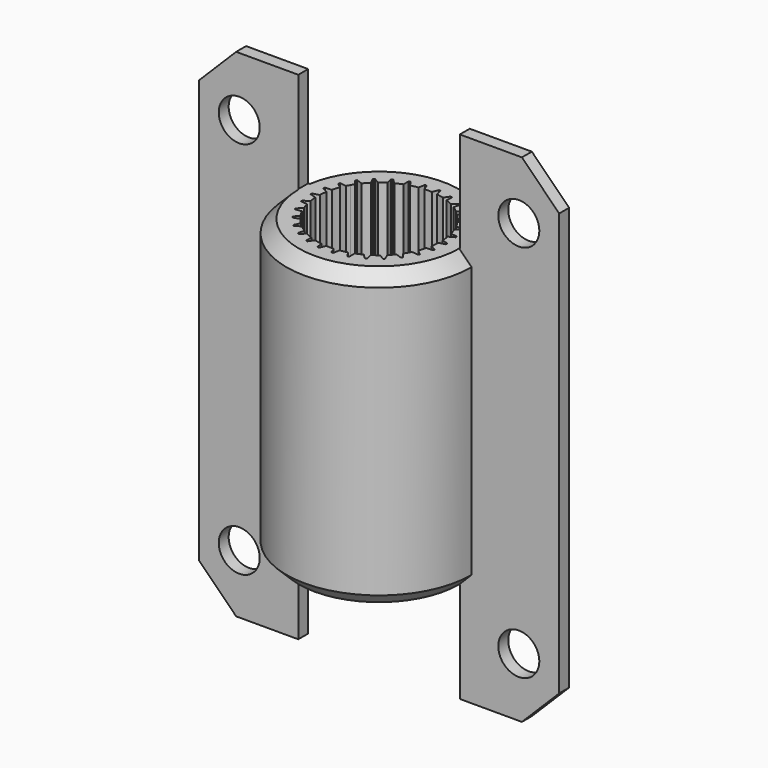
from build123d import *

# Parameters (mm, degrees)
F0_R         = 7.45
F1_DEPTH     = 11.9
F2_R         = 1.65
F3_DEPTH     = 1
F4_T2_ANGLE  = 180
F4_T6_ANGLE  = 204.1813114707
F4_T9_ANGLE  = 180
F4_T13_ANGLE = 204.1813114707
F5_SIZE      = 3


# Not quite as in the source:
# - a fillet or chamfer that OpenCascade refuses, or shapes differently, is made with other operations: its cross-section is extruded or revolved along the edge and cut away or added


with BuildPart() as f1:
    # F0 (on Top) → F1 (new body, symmetric)
    with BuildSketch(Plane.XY):
        Circle(F0_R)
        with BuildLine():
            ThreePointArc((5.449550226, 0.0700166693), (5.4498875553, 0.0350090569), (5.45, 0))
            ThreePointArc((5.45, 0), (5.4498875553, -0.0350090569), (5.449550226, -0.0700166693))
            ThreePointArc((5.449550226, -0.0700166693), (5.4201443298, -0.5696801248), (5.3450217628, -1.0645385646))
            ThreePointArc((5.3450217628, -1.0645385646), (5.330904424, -1.133118715), (5.3159071946, -1.2015118387))
            ThreePointArc((5.3159071946, -1.2015118387), (5.1832580138, -1.6841426193), (5.0068902002, -2.152568355))
            ThreePointArc((5.0068902002, -2.152568355), (4.9788227442, -2.2167147048), (4.9499335102, -2.2804951754))
            ThreePointArc((4.9499335102, -2.2804951754), (4.7198384506, -2.725), (4.4499335102, -3.1465205792))
            ThreePointArc((4.4499335102, -3.1465205792), (4.4091426193, -3.203429625), (4.3676239789, -3.2598099298))
            ThreePointArc((4.3676239789, -3.2598099298), (4.0501392989, -3.6467618047), (3.6984933726, -4.0029547553))
            ThreePointArc((3.6984933726, -4.0029547553), (3.6467618047, -4.0501392989), (3.5944283217, -4.096655348))
            ThreePointArc((3.5944283217, -4.096655348), (3.203429625, -4.4091426193), (2.7854113273, -4.6844406003))
            ThreePointArc((2.7854113273, -4.6844406003), (2.725, -4.7198384506), (2.6641388987, -4.7544572696))
            ThreePointArc((2.6641388987, -4.7544572696), (2.2167147048, -4.9788227442), (1.7505934411, -5.1611939127))
            ThreePointArc((1.7505934411, -5.1611939127), (1.6841426193, -5.1832580138), (1.617413822, -5.204466594))
            ThreePointArc((1.617413822, -5.204466594), (1.133118715, -5.330904424), (0.6392662213, -5.4123782849))
            ThreePointArc((0.6392662213, -5.4123782849), (0.5696801248, -5.4201443298), (0.5, -5.4270157545))
            ThreePointArc((0.5, -5.4270157545), (0, -5.45), (-0.5, -5.4270157545))
            ThreePointArc((-0.5, -5.4270157545), (-0.5696801248, -5.4201443298), (-0.6392662213, -5.4123782849))
            ThreePointArc((-0.6392662213, -5.4123782849), (-1.133118715, -5.330904424), (-1.617413822, -5.204466594))
            ThreePointArc((-1.617413822, -5.204466594), (-1.6841426193, -5.1832580138), (-1.7505934411, -5.1611939127))
            ThreePointArc((-1.7505934411, -5.1611939127), (-2.2167147048, -4.9788227442), (-2.6641388987, -4.7544572696))
            ThreePointArc((-2.6641388987, -4.7544572696), (-2.725, -4.7198384506), (-2.7854113273, -4.6844406003))
            ThreePointArc((-2.7854113273, -4.6844406003), (-3.203429625, -4.4091426193), (-3.5944283217, -4.096655348))
            ThreePointArc((-3.5944283217, -4.096655348), (-3.6467618047, -4.0501392989), (-3.6984933726, -4.0029547553))
            ThreePointArc((-3.6984933726, -4.0029547553), (-4.0501392989, -3.6467618047), (-4.3676239789, -3.2598099298))
            ThreePointArc((-4.3676239789, -3.2598099298), (-4.4091426193, -3.203429625), (-4.4499335102, -3.1465205792))
            ThreePointArc((-4.4499335102, -3.1465205792), (-4.7198384506, -2.725), (-4.9499335102, -2.2804951754))
            ThreePointArc((-4.9499335102, -2.2804951754), (-4.9788227442, -2.2167147048), (-5.0068902002, -2.152568355))
            ThreePointArc((-5.0068902002, -2.152568355), (-5.1832580138, -1.6841426193), (-5.3159071946, -1.2015118387))
            ThreePointArc((-5.3159071946, -1.2015118387), (-5.330904424, -1.133118715), (-5.3450217628, -1.0645385646))
            ThreePointArc((-5.3450217628, -1.0645385646), (-5.4201443298, -0.5696801248), (-5.449550226, -0.0700166693))
            ThreePointArc((-5.449550226, -0.0700166693), (-5.45, 0), (-5.449550226, 0.0700166693))
            ThreePointArc((-5.449550226, 0.0700166693), (-5.4201443298, 0.5696801248), (-5.3450217628, 1.0645385646))
            ThreePointArc((-5.3450217628, 1.0645385646), (-5.330904424, 1.133118715), (-5.3159071946, 1.2015118387))
            ThreePointArc((-5.3159071946, 1.2015118387), (-5.1832580138, 1.6841426193), (-5.0068902002, 2.152568355))
            ThreePointArc((-5.0068902002, 2.152568355), (-4.9788227442, 2.2167147048), (-4.9499335102, 2.2804951754))
            ThreePointArc((-4.9499335102, 2.2804951754), (-4.7198384506, 2.725), (-4.4499335102, 3.1465205792))
            ThreePointArc((-4.4499335102, 3.1465205792), (-4.4091426193, 3.203429625), (-4.3676239789, 3.2598099298))
            ThreePointArc((-4.3676239789, 3.2598099298), (-4.0501392989, 3.6467618047), (-3.6984933726, 4.0029547553))
            ThreePointArc((-3.6984933726, 4.0029547553), (-3.6467618047, 4.0501392989), (-3.5944283217, 4.096655348))
            ThreePointArc((-3.5944283217, 4.096655348), (-3.203429625, 4.4091426193), (-2.7854113273, 4.6844406003))
            ThreePointArc((-2.7854113273, 4.6844406003), (-2.725, 4.7198384506), (-2.6641388987, 4.7544572696))
            ThreePointArc((-2.6641388987, 4.7544572696), (-2.2167147048, 4.9788227442), (-1.7505934411, 5.1611939127))
            ThreePointArc((-1.7505934411, 5.1611939127), (-1.6841426193, 5.1832580138), (-1.617413822, 5.204466594))
            ThreePointArc((-1.617413822, 5.204466594), (-1.133118715, 5.330904424), (-0.6392662213, 5.4123782849))
            ThreePointArc((-0.6392662213, 5.4123782849), (-0.5696801248, 5.4201443298), (-0.5, 5.4270157545))
            ThreePointArc((-0.5, 5.4270157545), (0, 5.45), (0.5, 5.4270157545))
            ThreePointArc((0.5, 5.4270157545), (0.5696801248, 5.4201443298), (0.6392662213, 5.4123782849))
            ThreePointArc((0.6392662213, 5.4123782849), (1.133118715, 5.330904424), (1.617413822, 5.204466594))
            ThreePointArc((1.617413822, 5.204466594), (1.6841426193, 5.1832580138), (1.7505934411, 5.1611939127))
            ThreePointArc((1.7505934411, 5.1611939127), (2.2167147048, 4.9788227442), (2.6641388987, 4.7544572696))
            ThreePointArc((2.6641388987, 4.7544572696), (2.725, 4.7198384506), (2.7854113273, 4.6844406003))
            ThreePointArc((2.7854113273, 4.6844406003), (3.203429625, 4.4091426193), (3.5944283217, 4.096655348))
            ThreePointArc((3.5944283217, 4.096655348), (3.6467618047, 4.0501392989), (3.6984933726, 4.0029547553))
            ThreePointArc((3.6984933726, 4.0029547553), (4.0501392989, 3.6467618047), (4.3676239789, 3.2598099298))
            ThreePointArc((4.3676239789, 3.2598099298), (4.4091426193, 3.203429625), (4.4499335102, 3.1465205792))
            ThreePointArc((4.4499335102, 3.1465205792), (4.7198384506, 2.725), (4.9499335102, 2.2804951754))
            ThreePointArc((4.9499335102, 2.2804951754), (4.9788227442, 2.2167147048), (5.0068902002, 2.152568355))
            ThreePointArc((5.0068902002, 2.152568355), (5.1832580138, 1.6841426193), (5.3159071946, 1.2015118387))
            ThreePointArc((5.3159071946, 1.2015118387), (5.330904424, 1.133118715), (5.3450217628, 1.0645385646))
            ThreePointArc((5.3450217628, 1.0645385646), (5.4201443298, 0.5696801248), (5.449550226, 0.0700166693))
        make_face(mode=Mode.SUBTRACT)
        with BuildLine():
            Line((-3.471065627, 3.5290513475), (-3.6984933726, 4.0029547553))
            ThreePointArc((-3.6984933726, 4.0029547553), (-4.0501392989, 3.6467618047), (-4.3676239789, 3.2598099298))
            Line((-4.3676239789, 3.2598099298), (-3.8725439908, 3.0831644522))
            ThreePointArc((-3.8725439908, 3.0831644522), (-3.7772917267, 3.1991510141), (-3.6785668861, 3.3121965015))
            ThreePointArc((-3.6785668861, 3.3121965015), (-3.5764602296, 3.4221969882), (-3.471065627, 3.5290513475))
        make_face()
        with BuildLine():
            Line((-4.1289455477, 2.7302579849), (-4.4499335102, 3.1465205792))
            ThreePointArc((-4.4499335102, 3.1465205792), (-4.7198384506, 2.725), (-4.9499335102, 2.2804951754))
            Line((-4.9499335102, 2.2804951754), (-4.4289455477, 2.2106427427))
            ThreePointArc((-4.4289455477, 2.2106427427), (-4.3598897363, 2.3438987792), (-4.2868257487, 2.475))
            ThreePointArc((-4.2868257487, 2.475), (-4.2098207549, 2.6038258797), (-4.1289455477, 2.7302579849))
        make_face()
        with BuildLine():
            Line((-2.6614834824, 4.1736082318), (-2.7854113273, 4.6844406003))
            ThreePointArc((-2.7854113273, 4.6844406003), (-3.203429625, 4.4091426193), (-3.5944283217, 4.096655348))
            Line((-3.5944283217, 4.096655348), (-3.146893679, 3.8209370805))
            ThreePointArc((-3.146893679, 3.8209370805), (-3.0296079432, 3.9145849985), (-2.9095369988, 4.0046341222))
            ThreePointArc((-2.9095369988, 4.0046341222), (-2.7867912306, 4.0910016667), (-2.6614834824, 4.1736082318))
        make_face()
        with BuildLine():
            Line((-1.7355817384, 4.6357584093), (-1.7505934411, 5.1611939127))
            ThreePointArc((-1.7505934411, 5.1611939127), (-2.2167147048, 4.9788227442), (-2.6641388987, 4.7544572696))
            Line((-2.6641388987, 4.7544572696), (-2.283709013, 4.3917164234))
            ThreePointArc((-2.283709013, 4.3917164234), (-2.149515755, 4.4589328341), (-2.0133463832, 4.5220500153))
            ThreePointArc((-2.0133463832, 4.5220500153), (-1.8753260823, 4.5810099416), (-1.7355817384, 4.6357584093))
        make_face()
        with BuildLine():
            Line((-0.7338267442, 4.8953036994), (-0.6392662213, 5.4123782849))
            ThreePointArc((-0.6392662213, 5.4123782849), (-1.133118715, 5.330904424), (-1.617413822, 5.204466594))
            Line((-1.617413822, 5.204466594), (-1.3207153047, 4.7705566849))
            ThreePointArc((-1.3207153047, 4.7705566849), (-1.1754794137, 4.8084039086), (-1.0291628695, 4.8418306236))
            ThreePointArc((-1.0291628695, 4.8418306236), (-0.8819001854, 4.8708060999), (-0.7338267442, 4.8953036994))
        make_face()
        with BuildLine():
            Line((0.3, 4.9409007276), (0.5, 5.4270157545))
            ThreePointArc((0.5, 5.4270157545), (0, 5.45), (-0.5, 5.4270157545))
            Line((-0.5, 5.4270157545), (-0.3, 4.9409007276))
            ThreePointArc((-0.3, 4.9409007276), (-0.1500689814, 4.947724659), (0, 4.95))
            ThreePointArc((0, 4.95), (0.1500689814, 4.947724659), (0.3, 4.9409007276))
        make_face()
        with BuildLine():
            Line((1.3207153047, 4.7705566849), (1.617413822, 5.204466594))
            ThreePointArc((1.617413822, 5.204466594), (1.133118715, 5.330904424), (0.6392662213, 5.4123782849))
            Line((0.6392662213, 5.4123782849), (0.7338267442, 4.8953036994))
            ThreePointArc((0.7338267442, 4.8953036994), (0.8819001854, 4.8708060999), (1.0291628695, 4.8418306236))
            ThreePointArc((1.0291628695, 4.8418306236), (1.1754794137, 4.8084039086), (1.3207153047, 4.7705566849))
        make_face()
        with BuildLine():
            Line((2.283709013, 4.3917164234), (2.6641388987, 4.7544572696))
            ThreePointArc((2.6641388987, 4.7544572696), (2.2167147048, 4.9788227442), (1.7505934411, 5.1611939127))
            Line((1.7505934411, 5.1611939127), (1.7355817384, 4.6357584093))
            ThreePointArc((1.7355817384, 4.6357584093), (1.8753260823, 4.5810099416), (2.0133463832, 4.5220500153))
            ThreePointArc((2.0133463832, 4.5220500153), (2.149515755, 4.4589328341), (2.283709013, 4.3917164234))
        make_face()
        with BuildLine():
            Line((3.146893679, 3.8209370805), (3.5944283217, 4.096655348))
            ThreePointArc((3.5944283217, 4.096655348), (3.203429625, 4.4091426193), (2.7854113273, 4.6844406003))
            Line((2.7854113273, 4.6844406003), (2.6614834824, 4.1736082318))
            ThreePointArc((2.6614834824, 4.1736082318), (2.7867912306, 4.0910016667), (2.9095369988, 4.0046341222))
            ThreePointArc((2.9095369988, 4.0046341222), (3.0296079432, 3.9145849985), (3.146893679, 3.8209370805))
        make_face()
        with BuildLine():
            Line((3.8725439908, 3.0831644522), (4.3676239789, 3.2598099298))
            ThreePointArc((4.3676239789, 3.2598099298), (4.0501392989, 3.6467618047), (3.6984933726, 4.0029547553))
            Line((3.6984933726, 4.0029547553), (3.471065627, 3.5290513475))
            ThreePointArc((3.471065627, 3.5290513475), (3.5764602296, 3.4221969882), (3.6785668861, 3.3121965015))
            ThreePointArc((3.6785668861, 3.3121965015), (3.7772917267, 3.1991510141), (3.8725439908, 3.0831644522))
        make_face()
        with BuildLine():
            Line((4.4289455477, 2.2106427427), (4.9499335102, 2.2804951754))
            ThreePointArc((4.9499335102, 2.2804951754), (4.7198384506, 2.725), (4.4499335102, 3.1465205792))
            Line((4.4499335102, 3.1465205792), (4.1289455477, 2.7302579849))
            ThreePointArc((4.1289455477, 2.7302579849), (4.2098207549, 2.6038258797), (4.2868257487, 2.475))
            ThreePointArc((4.2868257487, 2.475), (4.3598897363, 2.3438987792), (4.4289455477, 2.2106427427))
        make_face()
        with BuildLine():
            Line((4.7917809317, 1.2415053375), (5.3159071946, 1.2015118387))
            ThreePointArc((5.3159071946, 1.2015118387), (5.1832580138, 1.6841426193), (5.0068902002, 2.152568355))
            Line((5.0068902002, 2.152568355), (4.606370735, 1.8121392472))
            ThreePointArc((4.606370735, 1.8121392472), (4.6591919121, 1.6716550858), (4.7077297557, 1.5296341222))
            ThreePointArc((4.7077297557, 1.5296341222), (4.7519396433, 1.3862069204), (4.7917809317, 1.2415053375))
        make_face()
        with BuildLine():
            Line((4.9451924954, 0.2181081916), (5.449550226, 0.0700166693))
            ThreePointArc((5.449550226, 0.0700166693), (5.4201443298, 0.5696801248), (5.3450217628, 1.0645385646))
            Line((5.3450217628, 1.0645385646), (4.8824754175, 0.8148213288))
            ThreePointArc((4.8824754175, 0.8148213288), (4.9049340256, 0.6664249431), (4.9228833821, 0.5174158932))
            ThreePointArc((4.9228833821, 0.5174158932), (4.9363069856, 0.3679311674), (4.9451924954, 0.2181081916))
        make_face()
        with BuildLine():
            Line((-4.606370735, 1.8121392472), (-5.0068902002, 2.152568355))
            ThreePointArc((-5.0068902002, 2.152568355), (-5.1832580138, 1.6841426193), (-5.3159071946, 1.2015118387))
            Line((-5.3159071946, 1.2015118387), (-4.7917809317, 1.2415053375))
            ThreePointArc((-4.7917809317, 1.2415053375), (-4.7519396433, 1.3862069204), (-4.7077297557, 1.5296341222))
            ThreePointArc((-4.7077297557, 1.5296341222), (-4.6591919121, 1.6716550858), (-4.606370735, 1.8121392472))
        make_face()
        with BuildLine():
            Line((-4.8824754175, 0.8148213288), (-5.3450217628, 1.0645385646))
            ThreePointArc((-5.3450217628, 1.0645385646), (-5.4201443298, 0.5696801248), (-5.449550226, 0.0700166693))
            Line((-5.449550226, 0.0700166693), (-4.9451924954, 0.2181081916))
            ThreePointArc((-4.9451924954, 0.2181081916), (-4.9363069856, 0.3679311674), (-4.9228833821, 0.5174158932))
            ThreePointArc((-4.9228833821, 0.5174158932), (-4.9049340256, 0.6664249431), (-4.8824754175, 0.8148213288))
        make_face()
        with BuildLine():
            ThreePointArc((-5.449550226, -0.0700166693), (-5.4201443298, -0.5696801248), (-5.3450217628, -1.0645385646))
            Line((-5.3450217628, -1.0645385646), (-4.8824754175, -0.8148213288))
            ThreePointArc((-4.8824754175, -0.8148213288), (-4.9049340256, -0.6664249431), (-4.9228833821, -0.5174158932))
            ThreePointArc((-4.9228833821, -0.5174158932), (-4.9363069856, -0.3679311674), (-4.9451924954, -0.2181081916))
            Line((-4.9451924954, -0.2181081916), (-5.449550226, -0.0700166693))
        make_face()
        with BuildLine():
            ThreePointArc((-5.3159071946, -1.2015118387), (-5.1832580138, -1.6841426193), (-5.0068902002, -2.152568355))
            Line((-5.0068902002, -2.152568355), (-4.606370735, -1.8121392472))
            ThreePointArc((-4.606370735, -1.8121392472), (-4.6591919121, -1.6716550858), (-4.7077297557, -1.5296341222))
            ThreePointArc((-4.7077297557, -1.5296341222), (-4.7519396433, -1.3862069204), (-4.7917809317, -1.2415053375))
            Line((-4.7917809317, -1.2415053375), (-5.3159071946, -1.2015118387))
        make_face()
        with BuildLine():
            ThreePointArc((-4.9499335102, -2.2804951754), (-4.7198384506, -2.725), (-4.4499335102, -3.1465205792))
            Line((-4.4499335102, -3.1465205792), (-4.1289455477, -2.7302579849))
            ThreePointArc((-4.1289455477, -2.7302579849), (-4.2098207549, -2.6038258797), (-4.2868257487, -2.475))
            ThreePointArc((-4.2868257487, -2.475), (-4.3598897363, -2.3438987792), (-4.4289455477, -2.2106427427))
            Line((-4.4289455477, -2.2106427427), (-4.9499335102, -2.2804951754))
        make_face()
        with BuildLine():
            ThreePointArc((-4.3676239789, -3.2598099298), (-4.0501392989, -3.6467618047), (-3.6984933726, -4.0029547553))
            Line((-3.6984933726, -4.0029547553), (-3.471065627, -3.5290513475))
            ThreePointArc((-3.471065627, -3.5290513475), (-3.5764602296, -3.4221969882), (-3.6785668861, -3.3121965015))
            ThreePointArc((-3.6785668861, -3.3121965015), (-3.7772917267, -3.1991510141), (-3.8725439908, -3.0831644522))
            Line((-3.8725439908, -3.0831644522), (-4.3676239789, -3.2598099298))
        make_face()
        with BuildLine():
            ThreePointArc((-3.5944283217, -4.096655348), (-3.203429625, -4.4091426193), (-2.7854113273, -4.6844406003))
            Line((-2.7854113273, -4.6844406003), (-2.6614834824, -4.1736082318))
            ThreePointArc((-2.6614834824, -4.1736082318), (-2.7867912306, -4.0910016667), (-2.9095369988, -4.0046341222))
            ThreePointArc((-2.9095369988, -4.0046341222), (-3.0296079432, -3.9145849985), (-3.146893679, -3.8209370805))
            Line((-3.146893679, -3.8209370805), (-3.5944283217, -4.096655348))
        make_face()
        with BuildLine():
            ThreePointArc((-2.6641388987, -4.7544572696), (-2.2167147048, -4.9788227442), (-1.7505934411, -5.1611939127))
            Line((-1.7505934411, -5.1611939127), (-1.7355817384, -4.6357584093))
            ThreePointArc((-1.7355817384, -4.6357584093), (-1.8753260823, -4.5810099416), (-2.0133463832, -4.5220500153))
            ThreePointArc((-2.0133463832, -4.5220500153), (-2.149515755, -4.4589328341), (-2.283709013, -4.3917164234))
            Line((-2.283709013, -4.3917164234), (-2.6641388987, -4.7544572696))
        make_face()
        with BuildLine():
            ThreePointArc((-1.617413822, -5.204466594), (-1.133118715, -5.330904424), (-0.6392662213, -5.4123782849))
            Line((-0.6392662213, -5.4123782849), (-0.7338267442, -4.8953036994))
            ThreePointArc((-0.7338267442, -4.8953036994), (-0.8819001854, -4.8708060999), (-1.0291628695, -4.8418306236))
            ThreePointArc((-1.0291628695, -4.8418306236), (-1.1754794137, -4.8084039086), (-1.3207153047, -4.7705566849))
            Line((-1.3207153047, -4.7705566849), (-1.617413822, -5.204466594))
        make_face()
        with BuildLine():
            ThreePointArc((-0.5, -5.4270157545), (0, -5.45), (0.5, -5.4270157545))
            Line((0.5, -5.4270157545), (0.3, -4.9409007276))
            ThreePointArc((0.3, -4.9409007276), (0.1500689814, -4.947724659), (0, -4.95))
            ThreePointArc((0, -4.95), (-0.1500689814, -4.947724659), (-0.3, -4.9409007276))
            Line((-0.3, -4.9409007276), (-0.5, -5.4270157545))
        make_face()
        with BuildLine():
            ThreePointArc((0.6392662213, -5.4123782849), (1.133118715, -5.330904424), (1.617413822, -5.204466594))
            Line((1.617413822, -5.204466594), (1.3207153047, -4.7705566849))
            ThreePointArc((1.3207153047, -4.7705566849), (1.1754794137, -4.8084039086), (1.0291628695, -4.8418306236))
            ThreePointArc((1.0291628695, -4.8418306236), (0.8819001854, -4.8708060999), (0.7338267442, -4.8953036994))
            Line((0.7338267442, -4.8953036994), (0.6392662213, -5.4123782849))
        make_face()
        with BuildLine():
            ThreePointArc((1.7505934411, -5.1611939127), (2.2167147048, -4.9788227442), (2.6641388987, -4.7544572696))
            Line((2.6641388987, -4.7544572696), (2.283709013, -4.3917164234))
            ThreePointArc((2.283709013, -4.3917164234), (2.149515755, -4.4589328341), (2.0133463832, -4.5220500153))
            ThreePointArc((2.0133463832, -4.5220500153), (1.8753260823, -4.5810099416), (1.7355817384, -4.6357584093))
            Line((1.7355817384, -4.6357584093), (1.7505934411, -5.1611939127))
        make_face()
        with BuildLine():
            ThreePointArc((2.7854113273, -4.6844406003), (3.203429625, -4.4091426193), (3.5944283217, -4.096655348))
            Line((3.5944283217, -4.096655348), (3.146893679, -3.8209370805))
            ThreePointArc((3.146893679, -3.8209370805), (3.0296079432, -3.9145849985), (2.9095369988, -4.0046341222))
            ThreePointArc((2.9095369988, -4.0046341222), (2.7867912306, -4.0910016667), (2.6614834824, -4.1736082318))
            Line((2.6614834824, -4.1736082318), (2.7854113273, -4.6844406003))
        make_face()
        with BuildLine():
            ThreePointArc((3.6984933726, -4.0029547553), (4.0501392989, -3.6467618047), (4.3676239789, -3.2598099298))
            Line((4.3676239789, -3.2598099298), (3.8725439908, -3.0831644522))
            ThreePointArc((3.8725439908, -3.0831644522), (3.7772917267, -3.1991510141), (3.6785668861, -3.3121965015))
            ThreePointArc((3.6785668861, -3.3121965015), (3.5764602296, -3.4221969882), (3.471065627, -3.5290513475))
            Line((3.471065627, -3.5290513475), (3.6984933726, -4.0029547553))
        make_face()
        with BuildLine():
            ThreePointArc((4.4499335102, -3.1465205792), (4.7198384506, -2.725), (4.9499335102, -2.2804951754))
            Line((4.9499335102, -2.2804951754), (4.4289455477, -2.2106427427))
            ThreePointArc((4.4289455477, -2.2106427427), (4.3598897363, -2.3438987792), (4.2868257487, -2.475))
            ThreePointArc((4.2868257487, -2.475), (4.2098207549, -2.6038258797), (4.1289455477, -2.7302579849))
            Line((4.1289455477, -2.7302579849), (4.4499335102, -3.1465205792))
        make_face()
        with BuildLine():
            ThreePointArc((5.0068902002, -2.152568355), (5.1832580138, -1.6841426193), (5.3159071946, -1.2015118387))
            Line((5.3159071946, -1.2015118387), (4.7917809317, -1.2415053375))
            ThreePointArc((4.7917809317, -1.2415053375), (4.7519396433, -1.3862069204), (4.7077297557, -1.5296341222))
            ThreePointArc((4.7077297557, -1.5296341222), (4.6591919121, -1.6716550858), (4.606370735, -1.8121392472))
            Line((4.606370735, -1.8121392472), (5.0068902002, -2.152568355))
        make_face()
        with BuildLine():
            ThreePointArc((5.3450217628, -1.0645385646), (5.4201443298, -0.5696801248), (5.449550226, -0.0700166693))
            Line((5.449550226, -0.0700166693), (4.9451924954, -0.2181081916))
            ThreePointArc((4.9451924954, -0.2181081916), (4.9363069856, -0.3679311674), (4.9228833821, -0.5174158932))
            ThreePointArc((4.9228833821, -0.5174158932), (4.9049340256, -0.6664249431), (4.8824754175, -0.8148213288))
            Line((4.8824754175, -0.8148213288), (5.3450217628, -1.0645385646))
        make_face()
    extrude(amount=F1_DEPTH, both=True)

    # F2 (on Front) → F3 (join)
    with BuildSketch(Plane.XZ):
        Polygon((-14.5, 0), (-14.5, -20), (-6.5, -20), (-6.5, 20), (-14.5, 20), align=None)
        with Locations((-11.25, -15.25)):
            Circle(F2_R, mode=Mode.SUBTRACT)
        with Locations((-11.25, 15.25)):
            Circle(F2_R, mode=Mode.SUBTRACT)
        Polygon((6.5, 20), (6.5, -20), (14.5, -20), (14.5, 0), (14.5, 20), align=None)
        with Locations((11.25, -15.25)):
            Circle(F2_R, mode=Mode.SUBTRACT)
        with Locations((11.25, 15.25)):
            Circle(F2_R, mode=Mode.SUBTRACT)
    extrude(amount=-F3_DEPTH)

    # F4: chamfer of 1 on 4 edges, made by hand

    # F4_s1 → F4_t2 (revolve, cut)
    with BuildSketch(Plane.XZ):
        with BuildLine():
            Line((-6.4217157288, -11.9282842712), (-7.4782842712, -10.8717157288))
            Line((-7.4782842712, -10.8717157288), (-7.4982842712, -10.8717157288))
            ThreePointArc((-7.4982842712, -10.8717157288), (-7.47, -11.3858578644), (-7.47, -11.9))
            Line((-7.47, -11.9), (-7.45, -11.92))
            ThreePointArc((-7.45, -11.92), (-6.9358578644, -11.92), (-6.4217157288, -11.9482842712))
            Line((-6.4217157288, -11.9482842712), (-6.4217157288, -11.9282842712))
        make_face()
    revolve(axis=Axis((0, 0, -11.9), (0, 0, 1)), revolution_arc=F4_T2_ANGLE, mode=Mode.SUBTRACT)


with BuildPart() as f4_tool4:
    # F4_s5 → F4_t6 (revolve)
    with BuildSketch(Plane(origin=(0, 0, 0), x_dir=(0, 0, 1), z_dir=(-0.2094590952, -0.9778174101, 0))):
        with BuildLine():
            Line((-11.9282842712, -6.4217157288), (-10.8717157288, -7.4782842712))
            Line((-10.8717157288, -7.4782842712), (-10.8717157288, -7.4982842712))
            ThreePointArc((-10.8717157288, -7.4982842712), (-11.3858578644, -7.47), (-11.9, -7.47))
            Line((-11.9, -7.47), (-11.92, -7.45))
            ThreePointArc((-11.92, -7.45), (-11.92, -6.9358578644), (-11.9482842712, -6.4217157288))
            Line((-11.9482842712, -6.4217157288), (-11.9282842712, -6.4217157288))
        make_face()
    revolve(axis=Axis((0, 0, -11.9), (0, 0, 1)), revolution_arc=F4_T6_ANGLE)

    split(bisect_by=Plane.XZ.offset(-1), keep=Keep.BOTTOM)


with BuildPart() as f1_1:
    add(f1.part)

    # F4_t3: cut F4_tool4
    add(f4_tool4.part, mode=Mode.SUBTRACT)

    # F4_s8 → F4_t9 (revolve, cut)
    with BuildSketch(Plane.XZ):
        with BuildLine():
            Line((-6.4217157288, 11.9282842712), (-7.4782842712, 10.8717157288))
            Line((-7.4782842712, 10.8717157288), (-7.4982842712, 10.8717157288))
            ThreePointArc((-7.4982842712, 10.8717157288), (-7.47, 11.3858578644), (-7.47, 11.9))
            Line((-7.47, 11.9), (-7.45, 11.92))
            ThreePointArc((-7.45, 11.92), (-6.9358578644, 11.92), (-6.4217157288, 11.9482842712))
            Line((-6.4217157288, 11.9482842712), (-6.4217157288, 11.9282842712))
        make_face()
    revolve(axis=Axis((0, 0, 11.9), (0, 0, 1)), revolution_arc=F4_T9_ANGLE, mode=Mode.SUBTRACT)


with BuildPart() as f4_tool11:
    # F4_s12 → F4_t13 (revolve)
    with BuildSketch(Plane(origin=(0, 0, 0), x_dir=(0, 0, 1), z_dir=(-0.2094590952, -0.9778174101, 0))):
        with BuildLine():
            Line((11.9282842712, -6.4217157288), (10.8717157288, -7.4782842712))
            Line((10.8717157288, -7.4782842712), (10.8717157288, -7.4982842712))
            ThreePointArc((10.8717157288, -7.4982842712), (11.3858578644, -7.47), (11.9, -7.47))
            Line((11.9, -7.47), (11.92, -7.45))
            ThreePointArc((11.92, -7.45), (11.92, -6.9358578644), (11.9482842712, -6.4217157288))
            Line((11.9482842712, -6.4217157288), (11.9282842712, -6.4217157288))
        make_face()
    revolve(axis=Axis((0, 0, 11.9), (0, 0, 1)), revolution_arc=F4_T13_ANGLE)

    split(bisect_by=Plane.XZ.offset(-1), keep=Keep.BOTTOM)


with BuildPart() as f1_2:
    add(f1_1.part)

    # F4_t10: cut F4_tool11
    add(f4_tool11.part, mode=Mode.SUBTRACT)

    # F5
    f5_edges = [f1_2.edges().sort_by_distance(p)[0] for p in [
        (-14.5, 0.5, 20),
        (14.5, 0.5, 20),
        (14.5, 0.5, -20),
        (-14.5, 0.5, -20),
    ]]
    chamfer(f5_edges, length=F5_SIZE)


solid = f1_2.part
